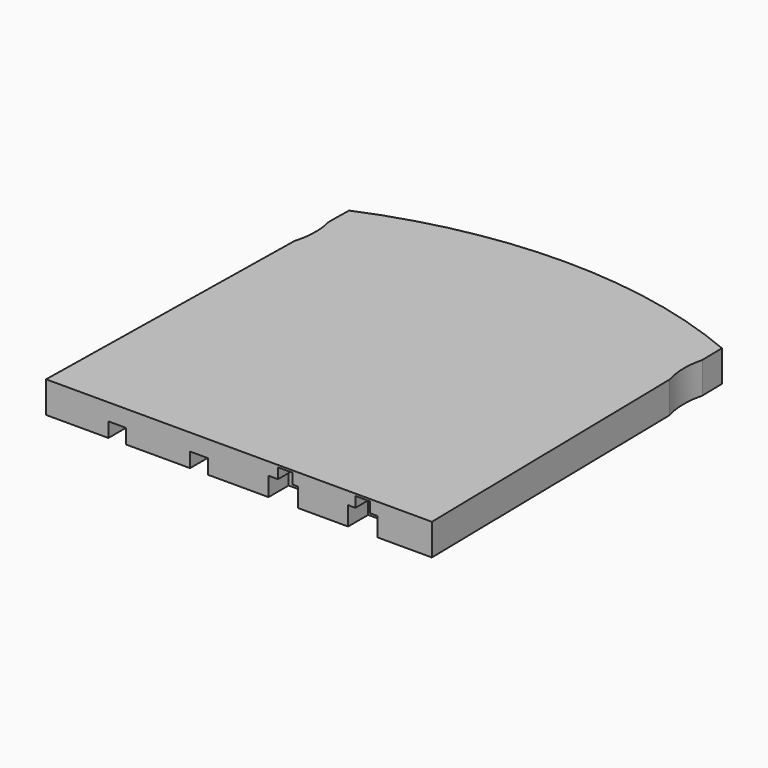
from build123d import *

# Parameters (mm, degrees)
F1_DEPTH      = 1.5
F2_R          = 1.8
F3_DEPTH      = 1.2
F5_DEPTH      = 1
F6_W          = 0.85
F6_H          = 2.5
F7_DEPTH      = 0.7
F8_W          = 0.7
F8_H          = 0.9
F9_DEPTH      = 1.2
F10_W         = 0.3
F10_H         = 0.3
F11_DEPTH     = 0.9
F12_TEXT_SIZE = 7.9904652421
F13_DEPTH     = 0.5


# Not quite as in the source:
# - Text() gives the source's letters only with a copy of the font that has no kerning and outlines rounded to 1/6400 em; it was checked with that copy


with BuildPart() as f1:
    # F0 (on Top) → F1 (new body)
    with BuildSketch(Plane.XY):
        with BuildLine():
            Line((-8.9560451977, 14.5), (-9.21, 0))
            Line((-9.21, 0), (9.21, 0))
            Line((9.21, 0), (8.9560451977, 14.5))
            ThreePointArc((8.9560451977, 14.5), (8.8000416812, 15.4975744796), (8.9210169492, 16.5))
            Line((8.9210169492, 16.5), (8.9, 17.7))
            Line((8.9, 17.7), (-8.9, 17.7))
            Line((-8.9, 17.7), (-8.9210169492, 16.5))
            ThreePointArc((-8.9210169492, 16.5), (-8.8000416812, 15.4975744796), (-8.9560451977, 14.5))
        make_face()
        with BuildLine():
            ThreePointArc((8.9, 17.7), (0, 19.5), (-8.9, 17.7))
            Line((-8.9, 17.7), (8.9, 17.7))
        make_face()
    extrude(amount=F1_DEPTH)

    # F2 (on Top) → F3 (cut)
    with BuildSketch(Plane.XY):
        with Locations((5.55, 16.6)):
            Circle(F2_R)
        with Locations((-5.55, 16.6)):
            Circle(F2_R)
    extrude(amount=F3_DEPTH, mode=Mode.SUBTRACT)

    # F4 (on face) → F5 (cut)
    with BuildSketch(Plane(origin=(0, 0, 0), x_dir=(1, 0, 0), z_dir=(0, 0, -1))):
        Polygon((-9.124180791, -4.9), (-0.51, -4.9), (-0.51, -2.5), (-9.1662146893, -2.5), align=None)
    extrude(amount=-F5_DEPTH, mode=Mode.SUBTRACT)

    # F6 (on face) → F7 (cut)
    with BuildSketch(Plane(origin=(0, 0, 0), x_dir=(1, 0, 0), z_dir=(0, 0, -1))):
        with Locations((-1.91, -1.25)):
            Rectangle(F6_W, F6_H)
        with Locations((-5.81, -1.25)):
            Rectangle(F6_W, F6_H)
    extrude(amount=-F7_DEPTH, mode=Mode.SUBTRACT)

    # F8 (on face) → F9 (cut)
    with BuildSketch(Plane.XZ):
        with Locations((6.26, 0.45)):
            Rectangle(F8_W, F8_H)
        with Locations((5.56, 0.45)):
            Rectangle(F8_W, F8_H)
        with Locations((1.76, 0.45)):
            Rectangle(F8_W, F8_H)
        with Locations((2.46, 0.45)):
            Rectangle(F8_W, F8_H)
    extrude(amount=-F9_DEPTH, mode=Mode.SUBTRACT)

    # F10 (on face) → F11 (cut)
    with BuildSketch(Plane.XZ):
        with Locations((2.21, 1.05)):
            Rectangle(F10_W, F10_H)
        Polygon((2.06, 0.9), (1.86, 0.9), (1.86, 0.7), (2.56, 0.7), (2.56, 0.9), (2.36, 0.9), align=None)
        Polygon((1.86, 1.4), (1.86, 0.9), (2.06, 0.9), (2.06, 1.2), (2.36, 1.2), (2.36, 0.9), (2.56, 0.9), (2.56, 1.4), align=None)
        Polygon((5.56, 1.4), (5.56, 0.9), (5.76, 0.9), (5.76, 1.2), (6.06, 1.2), (6.06, 0.9), (6.26, 0.9), (6.26, 1.4), align=None)
        with Locations((5.91, 1.05)):
            Rectangle(F10_W, F10_H)
        Polygon((5.76, 0.9), (5.56, 0.9), (5.56, 0.7), (6.26, 0.7), (6.26, 0.9), (6.06, 0.9), align=None)
    extrude(amount=-F11_DEPTH, mode=Mode.SUBTRACT)

    # F12 (on face) → F13 (cut)
    with BuildSketch(Plane(origin=(0, 0, 0), x_dir=(1, 0, 0), z_dir=(0, 0, -1))):
        with Locations((-4.0314394167, -13.5603129991)):
            Text('V1', F12_TEXT_SIZE, font='Open Sans', text_align=(TextAlign.LEFT, TextAlign.BOTTOM))
    extrude(amount=-F13_DEPTH, mode=Mode.SUBTRACT)


solid = f1.part
